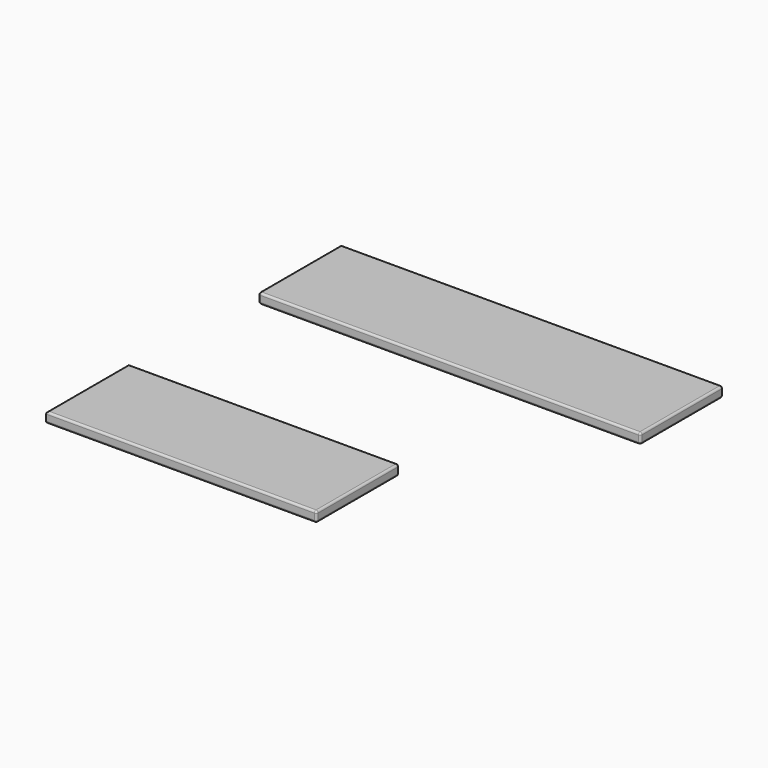
from build123d import *

# Parameters (mm, degrees)
F0_W     = 655
F0_H     = 250
F1_DEPTH = 25
F3_DEPTH = 250.001
F4_R     = 5
F5_W     = 925
F5_H     = 250
F6_DEPTH = 25
F7_R     = 5


with BuildPart() as f1:
    # F0 (on Top) → F1 (new body)
    with BuildSketch(Plane.XY):
        with Locations((46.5359067917, -735.1017089717)):
            Rectangle(F0_W, F0_H)
    extrude(amount=F1_DEPTH)

    # F2 (on face) → F3 (cut, through all)
    with BuildSketch(Plane.XZ.offset(860.1017089717)):
        Polygon((-329.5351266861, 5.0213485956), (-321.2029933929, 5.0213038921), (-293.8260436058, 27.9015563428), (-329.5351266861, 27.9015563428), align=None)
    extrude(amount=-F3_DEPTH, mode=Mode.SUBTRACT)

    # F4
    f4_edges = [f1.edges().sort_by_distance(p)[0] for p in [
        (46.535907, -610.101709, 25),
        (-280.964093, -735.101709, 25),
        (46.535907, -860.101709, 25),
        (374.035907, -735.101709, 25),
        (46.535907, -610.101709, 0),
        (-280.964093, -735.101709, 0),
        (46.535907, -860.101709, 0),
        (374.035907, -735.101709, 0),
        (374.035907, -860.101709, 12.5),
        (374.035907, -610.101709, 12.5),
    ]]
    fillet(f4_edges, radius=F4_R)


with BuildPart() as f6:
    # F5 (on Top) → F6 (new body)
    with BuildSketch(Plane.XY):
        with Locations((189.8969432941, -102.2657254338)):
            Rectangle(F5_W, F5_H)
    extrude(amount=F6_DEPTH)

    # F7
    f7_edges = [f6.edges().sort_by_distance(p)[0] for p in [
        (189.896943, 22.734275, 25),
        (-272.603057, -102.265725, 25),
        (189.896943, -227.265725, 25),
        (652.396943, -102.265725, 25),
        (189.896943, 22.734275, 0),
        (-272.603057, -102.265725, 0),
        (189.896943, -227.265725, 0),
        (652.396943, -102.265725, 0),
        (652.396943, 22.734275, 12.5),
        (-272.603057, 22.734275, 12.5),
        (-272.603057, -227.265725, 12.5),
        (652.396943, -227.265725, 12.5),
    ]]
    fillet(f7_edges, radius=F7_R)


solid = Compound([f1.part, f6.part])
